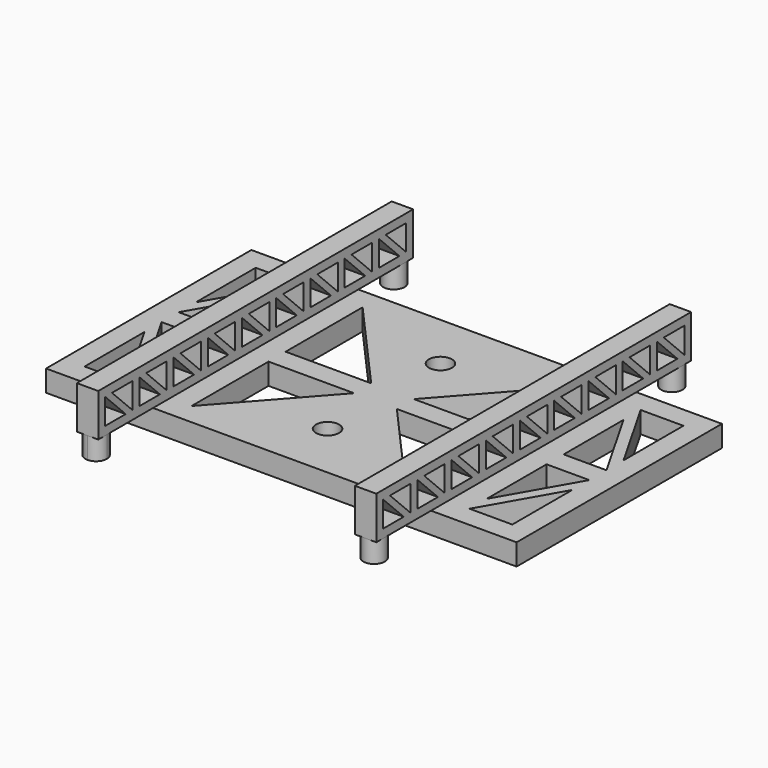
from build123d import *

# Parameters (mm, degrees)
F0_W     = 139.7
F0_H     = 76.2
F0_R     = 3.429
F1_DEPTH = 6.35
F2_W     = 6.35
F2_H     = 20.32
F2_H_2   = 76.2
F3_DEPTH = 12.7
F5_DEPTH = 114.301
F6_R     = 3.175
F7_DEPTH = 6.35


# Not quite as in the source:
# - a feature names something its author has since deleted; it is built from what else it names


with BuildPart() as f1:
    # F0 (on Top) → F1 (new body)
    with BuildSketch(Plane.XY):
        Rectangle(F0_W, F0_H)
        Polygon((-63.5, -9.525), (-50.8, -31.75), (-63.5, -31.75), align=None, mode=Mode.SUBTRACT)
        Polygon((-50.8, -25.4), (-63.5, -3.175), (-50.8, -3.175), align=None, mode=Mode.SUBTRACT)
        Polygon((-31.75, -31.75), (-31.75, -3.175), (-6.35, -3.175), align=None, mode=Mode.SUBTRACT)
        with Locations((0, -20.955)):
            Circle(F0_R, mode=Mode.SUBTRACT)
        Polygon((50.8, -31.75), (63.5, -9.525), (63.5, -31.75), align=None, mode=Mode.SUBTRACT)
        Polygon((31.75, -31.75), (6.35, -3.175), (31.75, -3.175), align=None, mode=Mode.SUBTRACT)
        Polygon((63.5, -3.175), (50.8, -25.4), (50.8, -3.175), align=None, mode=Mode.SUBTRACT)
        Polygon((-50.8, 25.4), (-50.8, 3.175), (-63.5, 3.175), align=None, mode=Mode.SUBTRACT)
        Polygon((-6.35, 3.175), (-31.75, 3.175), (-31.75, 31.75), align=None, mode=Mode.SUBTRACT)
        Polygon((-50.8, 31.75), (-63.5, 9.525), (-63.5, 31.75), align=None, mode=Mode.SUBTRACT)
        Polygon((6.35, 3.175), (31.75, 31.75), (31.75, 3.175), align=None, mode=Mode.SUBTRACT)
        Polygon((63.5, 3.175), (50.8, 3.175), (50.8, 25.4), align=None, mode=Mode.SUBTRACT)
        with Locations((0, 20.955)):
            Circle(F0_R, mode=Mode.SUBTRACT)
        Polygon((63.5, 9.525), (50.8, 31.75), (63.5, 31.75), align=None, mode=Mode.SUBTRACT)
    extrude(amount=F1_DEPTH)

    # F2 (on face) → F3 (join)
    with BuildSketch(Plane.XY.offset(6.35)):
        with Locations((41.275, -48.26)):
            Rectangle(F2_W, F2_H)
        with Locations((41.275, 0)):
            Rectangle(F2_W, F2_H_2)
        with Locations((41.275, 48.26)):
            Rectangle(F2_W, F2_H)
        with Locations((-41.275, 48.26)):
            Rectangle(F2_W, F2_H)
        with Locations((-41.275, 0)):
            Rectangle(F2_W, F2_H_2)
        with Locations((-41.275, -48.26)):
            Rectangle(F2_W, F2_H)
    extrude(amount=F3_DEPTH)

    # F4 (on face) → F5 (cut, through all)
    with BuildSketch(Plane.YZ.offset(44.45)):
        Polygon((-48.26, 8.89), (-55.88, 16.51), (-55.88, 8.89), align=None)
        Polygon((-45.72, 16.51), (-53.34, 16.51), (-45.72, 8.89), align=None)
        Polygon((-40.64, 16.51), (-33.02, 8.89), (-33.02, 16.51), align=None)
        Polygon((-43.18, 8.89), (-35.56, 8.89), (-43.18, 16.51), align=None)
        Polygon((-27.94, 16.51), (-20.32, 8.89), (-20.32, 16.51), align=None)
        Polygon((-30.48, 8.89), (-22.86, 8.89), (-30.48, 16.51), align=None)
        Polygon((-15.24, 16.51), (-7.62, 8.89), (-7.62, 16.51), align=None)
        Polygon((-17.78, 8.89), (-10.16, 8.89), (-17.78, 16.51), align=None)
        Polygon((-2.54, 16.51), (5.08, 8.89), (5.08, 16.51), align=None)
        Polygon((-5.08, 8.89), (2.54, 8.89), (-5.08, 16.51), align=None)
        Polygon((10.16, 16.51), (17.78, 8.89), (17.78, 16.51), align=None)
        Polygon((7.62, 8.89), (15.24, 8.89), (7.62, 16.51), align=None)
        Polygon((22.86, 16.51), (30.48, 8.89), (30.48, 16.51), align=None)
        Polygon((20.32, 8.89), (27.94, 8.89), (20.32, 16.51), align=None)
        Polygon((35.56, 16.51), (43.18, 8.89), (43.18, 16.51), align=None)
        Polygon((33.02, 8.89), (40.64, 8.89), (33.02, 16.51), align=None)
        Polygon((48.26, 16.51), (55.88, 8.89), (55.88, 16.51), align=None)
        Polygon((45.72, 8.89), (53.34, 8.89), (45.72, 16.51), align=None)
    extrude(amount=-F5_DEPTH, mode=Mode.SUBTRACT)

    # F6 (on face) → F7 (join)
    with BuildSketch(Plane(origin=(0, 0, 6.35), x_dir=(1, 0, 0), z_dir=(0, 0, -1))):
        with BuildLine():
            ThreePointArc((-44.45, 55.245), (-41.275, 52.07), (-38.1, 55.245))
            ThreePointArc((-38.1, 55.245), (-39.0299359697, 57.4900640303), (-41.275, 58.42))
            ThreePointArc((-41.275, 58.42), (-43.5200640303, 57.4900640303), (-44.45, 55.245))
        make_face()
        with Locations((41.275, 55.245)):
            Circle(F6_R)
        with Locations((-41.275, -55.245)):
            Circle(F6_R)
        with Locations((41.275, -55.245)):
            Circle(F6_R)
    extrude(amount=F7_DEPTH)


solid = f1.part
